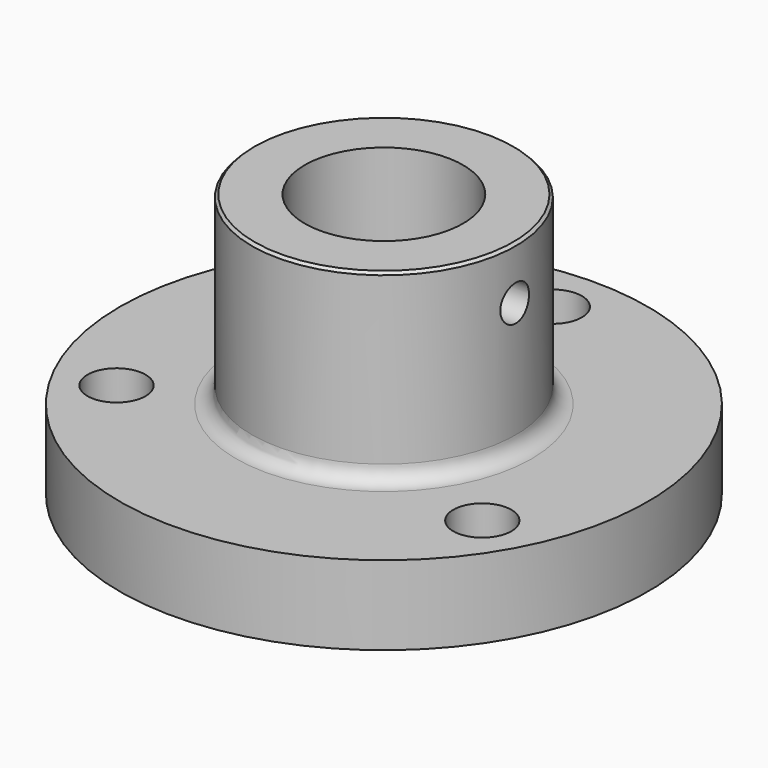
from build123d import *

# Parameters (mm, degrees)
F2_R            = 3
F4_D            = 6.8
F4_DEPTH        = 50.001
F5_R            = 5.5
F6_DEPTH        = 15.001
F6_COPIES_COUNT = 3
F7_SIZE         = 0.5


# Not quite as in the source:
# - a pattern or mirror of a feature is missing from the dataset's text; its kind, count and spacing are read off the source's solid


with BuildPart() as f1:
    # F0 (on Front) → F1 (revolve)
    with BuildSketch(Plane.XZ):
        Polygon((-15, 4), (-15, 50), (-25, 50), (-25, 15), (-50, 15), (-50, 0), (-20, 0), (-20, 4), align=None)
    revolve(axis=Axis((0, 0, 33.7237479181), (0, 0, 1)))

    # F2
    f2_edges = [f1.edges().sort_by_distance(p)[0] for p in [
        (25, 0, 15),
    ]]
    fillet(f2_edges, radius=F2_R)

    # F4 (through all, one way)
    with BuildSketch(Plane(origin=(0, 0, 0), x_dir=(0, 1, 0), z_dir=(-1, 0, 0))):
        with Locations((0, -40)):
            Circle(F4_D / 2)
    extrude(amount=-F4_DEPTH, mode=Mode.SUBTRACT)

    # F5 (on face) → F6 (cut, through all)
    with BuildSketch(Plane.XY.offset(15)):
        with Locations((0, 40)):
            Circle(F5_R)
    f6 = extrude(amount=-F6_DEPTH, mode=Mode.SUBTRACT)

    # F6_copies: F6 ×3 about axis
    f6_copies_axis = Axis((0, 0, 0), (0, 0, 1))
    for i in range(1, F6_COPIES_COUNT):
        add(f6.rotate(f6_copies_axis, i * 360 / F6_COPIES_COUNT), mode=Mode.SUBTRACT)

    # F7
    f7_edges = [f1.edges().sort_by_distance(p)[0] for p in [
        (25, 0, 50),
    ]]
    chamfer(f7_edges, length=F7_SIZE)


solid = f1.part
